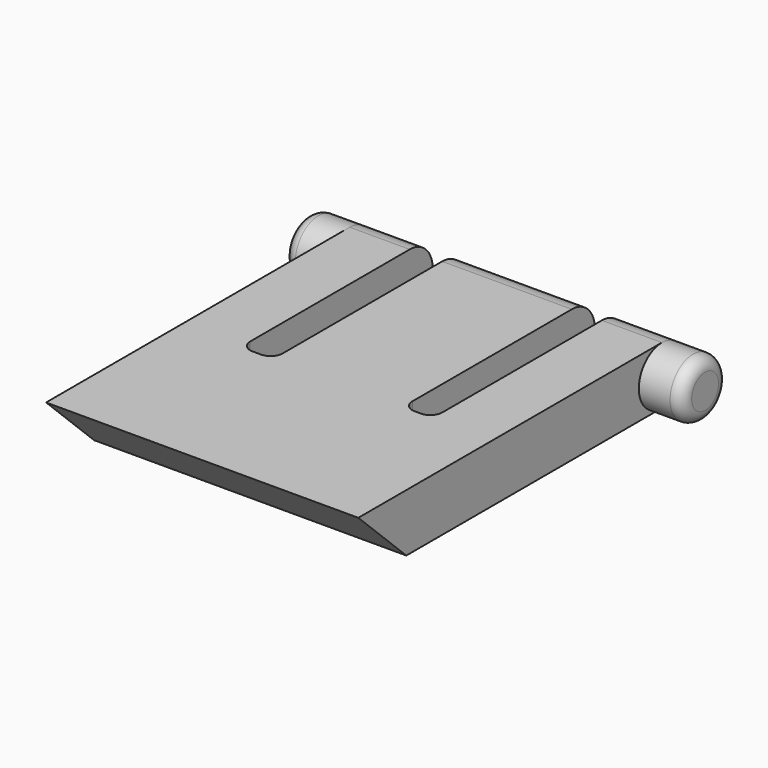
from build123d import *

# Parameters (mm, degrees)
F0_W      = 16.51
F0_H      = 21.59
F1_DEPTH  = 3.048
F2_W      = 1.7145
F2_H      = 12.7
F3_DEPTH  = 25.4
F4_W      = 1.5875
F4_H      = 12.7
F5_DEPTH  = 25.4
F7_DEPTH  = 25.4
F8_R      = 1.52399
F9_R      = 1.524
F10_DEPTH = 2.286
F11_R     = 1.524
F12_DEPTH = 2.286
F13_R     = 0.635
F14_R     = 0.635


# Not quite as in the source:
# - a fillet or chamfer is up to 0.001 mm smaller than in the source, because OpenCascade refuses the exact size


with BuildPart() as f1:
    # F0 (on Top) → F1 (new body)
    with BuildSketch(Plane.XY):
        with Locations((8.255, 10.795)):
            Rectangle(F0_W, F0_H)
    extrude(amount=F1_DEPTH)

    # F2 (on face) → F3 (cut)
    with BuildSketch(Plane.XY.offset(3.048)):
        with Locations((4.03225, 15.24)):
            Rectangle(F2_W, F2_H)
    extrude(amount=-F3_DEPTH, mode=Mode.SUBTRACT)

    # F4 (on face) → F5 (cut)
    with BuildSketch(Plane.XY.offset(3.048)):
        with Locations((12.54125, 15.24)):
            Rectangle(F4_W, F4_H)
    extrude(amount=-F5_DEPTH, mode=Mode.SUBTRACT)

    # F6 (on face) → F7 (cut)
    with BuildSketch(Plane(origin=(0, 0, 0), x_dir=(0, -1, 0), z_dir=(-1, 0, 0))):
        Polygon((0, 0), (0, 3.048), (-3.175, 0), align=None)
    extrude(amount=-F7_DEPTH, mode=Mode.SUBTRACT)

    # F8 (radius 1.524 in the source; OpenCascade refuses exactly that, so slightly less here)
    f8_edges = [f1.edges().sort_by_distance(p)[0] for p in [
        (1.5875, 21.59, 3.048),
        (1.5875, 21.59, 0),
        (8.3185, 21.59, 3.048),
        (8.3185, 21.59, 0),
        (14.9225, 21.59, 3.048),
        (14.9225, 21.59, 0),
    ]]
    fillet(f8_edges, radius=F8_R)

    # F9 (on face) → F10 (join)
    with BuildSketch(Plane(origin=(0, 0, 0), x_dir=(0, -1, 0), z_dir=(-1, 0, 0))):
        with Locations((-20.066, 1.524)):
            Circle(F9_R)
    extrude(amount=F10_DEPTH)

    # F11 (on face) → F12 (join)
    with BuildSketch(Plane.YZ.offset(16.51)):
        with Locations((20.066, 1.524)):
            Circle(F11_R)
    extrude(amount=F12_DEPTH)

    # F13
    f13_edges = [f1.edges().sort_by_distance(p)[0] for p in [
        (18.796, 18.542, 1.524),
        (-2.286, 21.59, 1.524),
    ]]
    fillet(f13_edges, radius=F13_R)

    # F14
    f14_edges = [f1.edges().sort_by_distance(p)[0] for p in [
        (11.7475, 8.89, 1.524),
        (13.335, 8.89, 1.524),
        (3.175, 8.89, 1.524),
        (4.8895, 8.89, 1.524),
    ]]
    fillet(f14_edges, radius=F14_R)


solid = f1.part
